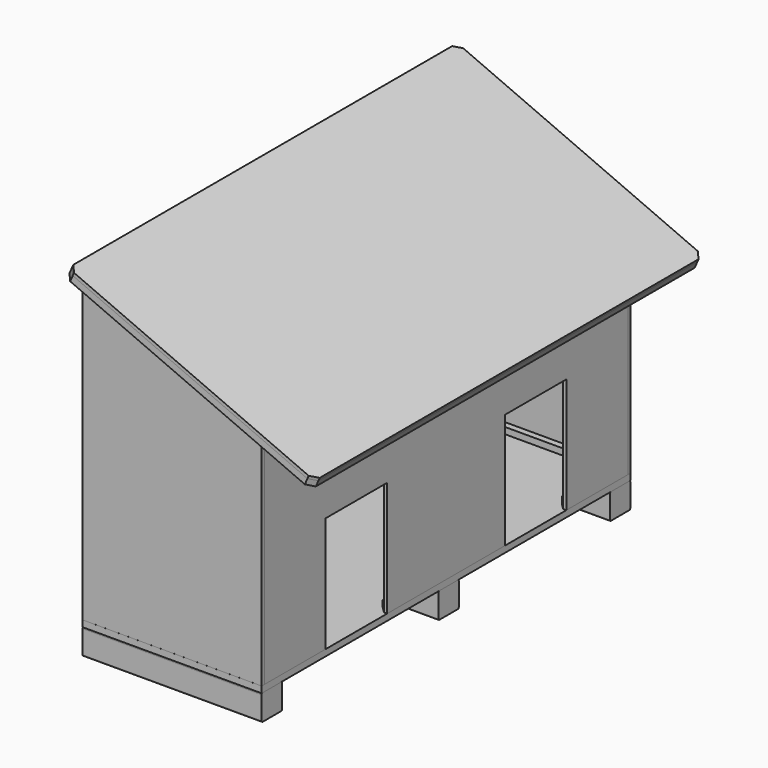
from build123d import *

# Parameters (mm, degrees)
F0_W      = 1803.4
F0_H      = 1219.2
F1_DEPTH  = 12.7
F3_DEPTH  = 12.7
F5_W      = 711.2
F5_H      = 1828.8
F6_DEPTH  = 25.4
F7_W      = 12.7
F7_H      = 901.7
F8_DEPTH  = 1803.4
F9_W      = 304.8
F9_H      = 457.2
F10_DEPTH = 12.7
F11_W     = 711.2
F11_H     = 101.6
F12_DEPTH = 101.6
F13_R     = 5.08
F16_W     = 25.4
F16_H     = 1219.2
F17_DEPTH = 25.4
F18_SIZE2 = 8.63599
F18_SIZE  = 25.39999
F20_W     = 1752.6
F20_H     = 25.4
F21_DEPTH = 25.4
F22_W     = 25.4
F22_H     = 927.1
F23_DEPTH = 25.4
F24_SIZE2 = 25.39999
F24_SIZE  = 8.63599
F26_W     = 279.4
F26_H     = 25.4
F27_DEPTH = 25.4
F28_SIZE  = 25.39999
F29_W     = 584.2
F29_H     = 25.4
F30_DEPTH = 25.4
F31_SIZE  = 25.39999
F32_W     = 279.4
F32_H     = 25.4
F33_DEPTH = 25.4
F34_SIZE  = 25.39999
F35_W     = 635
F35_H     = 25.4
F36_DEPTH = 25.4
F38_W     = 1066.8
F38_H     = 1930.4
F39_DEPTH = 12.7
F40_SIZE  = 25.4
F41_W     = 25.4
F41_H     = 1930.4
F42_DEPTH = 25.4
F43_SIZE  = 25.39999
F44_W     = 1041.4
F44_H     = 25.4
F45_DEPTH = 25.4
F46_SIZE  = 25.39999
F47_W     = 1041.4
F47_H     = 25.4
F48_DEPTH = 25.4
F49_SIZE  = 25.39999
F50_W     = 25.4
F50_H     = 1879.6
F51_DEPTH = 25.4
F53_DEPTH = 25.4
F55_W     = 101.6
F55_H     = 774.7
F56_DEPTH = 50.8


# Not quite as in the source:
# - a fillet or chamfer is up to 0.001 mm smaller than in the source, because OpenCascade refuses the exact size


with BuildPart() as f1:
    # F0 (on Right) → F1 (new body)
    with BuildSketch(Plane.YZ):
        with Locations((901.7, 609.6)):
            Rectangle(F0_W, F0_H)
    extrude(amount=F1_DEPTH)


with BuildPart() as f3:
    # F2 (on face) → F3 (new body)
    with BuildSketch(Plane(origin=(0, 1803.4, 0), x_dir=(-1, 0, 0), z_dir=(0, 1, 0))):
        Polygon((-711.2, 0), (0, 0), (0, 1219.2), (-12.7, 1219.2), (-711.2, 914.4), align=None)
    extrude(amount=F3_DEPTH)


with BuildPart() as f4_1:
    # F4: copy of F3
    add(f3.part.moved(Location((0, -1816.1, 0))))


with BuildPart() as f6:
    # F5 (on Top) → F6 (new body)
    with BuildSketch(Plane.XY):
        with Locations((355.6, 901.5832041594)):
            Rectangle(F5_W, F5_H)
    extrude(amount=-F6_DEPTH)


with BuildPart() as f8:
    # F7 (on face) → F8 (new body)
    with BuildSketch(Plane.XZ.offset(-1803.4)):
        with Locations((704.85, 450.85)):
            Rectangle(F7_W, F7_H)
    extrude(amount=F8_DEPTH)

    # F9 (on face) → F10 (cut)
    with BuildSketch(Plane.YZ.offset(711.2)):
        with Locations((457.2, 228.6)):
            Rectangle(F9_W, F9_H)
        with Locations((1346.2, 228.6)):
            Rectangle(F9_W, F9_H)
    extrude(amount=-F10_DEPTH, mode=Mode.SUBTRACT)


with BuildPart() as f12:
    # F11 (on face) → F12 (new body)
    with BuildSketch(Plane(origin=(0, 0, -25.4), x_dir=(1, 0, 0), z_dir=(0, 0, -1))):
        with Locations((355.6, -37.9832041594)):
            Rectangle(F11_W, F11_H)
    extrude(amount=F12_DEPTH)

    # F13
    f13_edges = [f12.edges().sort_by_distance(p)[0] for p in [
        (355.6, -12.816796, -127),
        (355.6, 88.783204, -127),
        (355.6, 88.783204, -25.4),
        (355.6, -12.816796, -25.4),
    ]]
    fillet(f13_edges, radius=F13_R)


with BuildPart() as f14_1:
    # F14: copy of F12
    add(f12.part.moved(Location((0, 876.3, 0))))


with BuildPart() as f15_1:
    # F15: copy of F12
    add(f12.part.moved(Location((0, 1727.2, 0))))


with BuildPart() as f17:
    # F16 (on face) → F17 (new body)
    with BuildSketch(Plane.YZ.offset(12.7)):
        with Locations((12.7, 609.6)):
            Rectangle(F16_W, F16_H)
    extrude(amount=F17_DEPTH)

    # F18 (size 25.4 and 8.636 in the source; OpenCascade refuses exactly that, so slightly less here)
    f18_edges = [f17.edges().sort_by_distance(p)[0] for p in [
        (38.1, 12.7, 1219.2),
    ]]
    f18_side = f17.faces().sort_by_distance((25.4, 12.7, 1219.2))[0]
    chamfer(f18_edges, length=F18_SIZE, length2=F18_SIZE2, reference=f18_side)


with BuildPart() as f19_1:
    # F19: copy of F17
    add(f17.part.moved(Location((0, 1778, 0))))


with BuildPart() as f21:
    # F20 (on face) → F21 (new body)
    with BuildSketch(Plane.YZ.offset(12.7)):
        with Locations((901.7, 12.7)):
            Rectangle(F20_W, F20_H)
    extrude(amount=F21_DEPTH)


with BuildPart() as f23:
    # F22 (on face) → F23 (new body)
    with BuildSketch(Plane(origin=(698.5, 0, 0), x_dir=(0, -1, 0), z_dir=(-1, 0, 0))):
        with Locations((-1790.7, 463.55)):
            Rectangle(F22_W, F22_H)
    extrude(amount=F23_DEPTH)

    # F24 (size 8.636 and 25.4 in the source; OpenCascade refuses exactly that, so slightly less here)
    f24_edges = [f23.edges().sort_by_distance(p)[0] for p in [
        (698.5, 1790.7, 927.1),
    ]]
    f24_side = f23.faces().sort_by_distance((698.5, 1790.7, 463.55))[0]
    chamfer(f24_edges, length=F24_SIZE, length2=F24_SIZE2, reference=f24_side)


with BuildPart() as f25_1:
    # F25: copy of F23
    add(f23.part.moved(Location((0, -1778, 0))))


with BuildPart() as f27:
    # F26 (on face) → F27 (new body)
    with BuildSketch(Plane(origin=(698.5, 0, 0), x_dir=(0, -1, 0), z_dir=(-1, 0, 0))):
        with Locations((-1638.3, 12.7)):
            Rectangle(F26_W, F26_H)
    extrude(amount=F27_DEPTH)

    # F28 (size 25.4 in the source; OpenCascade refuses exactly that, so slightly less here)
    f28_edges = [f27.edges().sort_by_distance(p)[0] for p in [
        (673.1, 1498.6, 12.7),
    ]]
    chamfer(f28_edges, length=F28_SIZE)


with BuildPart() as f30:
    # F29 (on face) → F30 (new body)
    with BuildSketch(Plane(origin=(698.5, 0, 0), x_dir=(0, -1, 0), z_dir=(-1, 0, 0))):
        with Locations((-901.7, 12.7)):
            Rectangle(F29_W, F29_H)
    extrude(amount=F30_DEPTH)

    # F31 (size 25.4 in the source; OpenCascade refuses exactly that, so slightly less here)
    f31_edges = [f30.edges().sort_by_distance(p)[0] for p in [
        (673.1, 1193.8, 12.7),
        (673.1, 609.6, 12.7),
    ]]
    chamfer(f31_edges, length=F31_SIZE)


with BuildPart() as f33:
    # F32 (on face) → F33 (new body)
    with BuildSketch(Plane(origin=(698.5, 0, 0), x_dir=(0, -1, 0), z_dir=(-1, 0, 0))):
        with Locations((-165.1, 12.7)):
            Rectangle(F32_W, F32_H)
    extrude(amount=F33_DEPTH)

    # F34 (size 25.4 in the source; OpenCascade refuses exactly that, so slightly less here)
    f34_edges = [f33.edges().sort_by_distance(p)[0] for p in [
        (673.1, 304.8, 12.7),
    ]]
    chamfer(f34_edges, length=F34_SIZE)


with BuildPart() as f36:
    # F35 (on face) → F36 (new body)
    with BuildSketch(Plane.XZ.offset(-1803.4)):
        with Locations((355.6, 12.7)):
            Rectangle(F35_W, F35_H)
    extrude(amount=F36_DEPTH)


with BuildPart() as f37_1:
    # F37: copy of F36
    add(f36.part.moved(Location((0, -1778, 0))))


with BuildPart() as f39:
    # F38 (on face) → F39 (new body)
    with BuildSketch(Plane(origin=(448.9472924188, 0, 1028.8375451264), x_dir=(0.9165393784, 0, -0.399944456), z_dir=(0.399944456, 0, 0.9165393784))):
        with Locations((20.3877192255, 901.7)):
            Rectangle(F38_W, F38_H)
    extrude(amount=F39_DEPTH)

    # F40
    f40_edges = [f39.edges().sort_by_distance(p)[0] for p in [
        (959.055192, -63.5, 813.173242),
        (959.055192, 1866.9, 813.173242),
        (-18.709017, 1866.9, 1239.833988),
        (-18.709017, -63.5, 1239.833988),
    ]]
    chamfer(f40_edges, length=F40_SIZE)


with BuildPart() as f42:
    # F41 (on face) → F42 (new body)
    with BuildSketch(Plane(origin=(448.9472924188, 0, 1028.8375451264), x_dir=(0.9165393784, 0, -0.399944456), z_dir=(-0.399944456, 0, -0.9165393784))):
        with Locations((-500.3122807745, -901.7)):
            Rectangle(F41_W, F41_H)
    extrude(amount=F42_DEPTH)

    # F43 (size 25.4 in the source; OpenCascade refuses exactly that, so slightly less here)
    f43_edges = [f42.edges().sort_by_distance(p)[0] for p in [
        (-26.327959, 1866.9, 1222.373913),
        (-26.327959, -63.5, 1222.373913),
    ]]
    chamfer(f43_edges, length=F43_SIZE)


with BuildPart() as f45:
    # F44 (on face) → F45 (new body)
    with BuildSketch(Plane(origin=(448.9472924188, 0, 1028.8375451264), x_dir=(0.9165393784, 0, -0.399944456), z_dir=(-0.399944456, 0, -0.9165393784))):
        with Locations((33.0877192255, -1854.2)):
            Rectangle(F44_W, F44_H)
    extrude(amount=F45_DEPTH)

    # F46 (size 25.4 in the source; OpenCascade refuses exactly that, so slightly less here)
    f46_edges = [f45.edges().sort_by_distance(p)[0] for p in [
        (951.43625, 1866.9, 795.713167),
    ]]
    chamfer(f46_edges, length=F46_SIZE)


with BuildPart() as f48:
    # F47 (on face) → F48 (new body)
    with BuildSketch(Plane(origin=(448.9472924188, 0, 1028.8375451264), x_dir=(0.9165393784, 0, -0.399944456), z_dir=(-0.399944456, 0, -0.9165393784))):
        with Locations((33.0877192255, 50.8)):
            Rectangle(F47_W, F47_H)
    extrude(amount=F48_DEPTH)

    # F49 (size 25.4 in the source; OpenCascade refuses exactly that, so slightly less here)
    f49_edges = [f48.edges().sort_by_distance(p)[0] for p in [
        (951.43625, -63.5, 795.713167),
    ]]
    chamfer(f49_edges, length=F49_SIZE)


with BuildPart() as f51:
    # F50 (on face) → F51 (new body)
    with BuildSketch(Plane(origin=(448.9472924188, 0, 1028.8375451264), x_dir=(0.9165393784, 0, -0.399944456), z_dir=(-0.399944456, 0, -0.9165393784))):
        with Locations((541.0877192255, -901.7)):
            Rectangle(F50_W, F50_H)
    extrude(amount=F51_DEPTH)


with BuildPart() as f53:
    # F52 (on face) → F53 (new body)
    with BuildSketch(Plane(origin=(0, 0, 0), x_dir=(-1, 0, 0), z_dir=(0, 1, 0))):
        Polygon((-673.1, 903.3125154187), (-38.1, 1180.4034245096), (-38.1, 1208.1163636364), (-673.1, 931.0254545455), align=None)
    extrude(amount=F53_DEPTH)


with BuildPart() as f54_1:
    # F54: copy of F53
    add(f53.part.moved(Location((0, 1778, 0))))


with BuildPart() as f56:
    # F55 (on face) → F56 (new body)
    with BuildSketch(Plane(origin=(0, 0, -25.4), x_dir=(1, 0, 0), z_dir=(0, 0, -1))):
        with Locations((495.3, -476.1332041594)):
            Rectangle(F55_W, F55_H)
    extrude(amount=F56_DEPTH)


with BuildPart() as f57_1:
    # F57: copy of F56
    add(f56.part.moved(Location((-279.4, 0, 0))))


with BuildPart() as f58_1:
    # F58: copy of F56
    add(f56.part.moved(Location((0, 863.6, 0))))


with BuildPart() as f59_1:
    # F59: copy of F57_1
    add(f57_1.part.moved(Location((0, 863.6, 0))))


solid = Compound([f1.part, f3.part, f4_1.part, f6.part, f8.part, f12.part, f14_1.part, f15_1.part, f17.part, f19_1.part, f21.part, f23.part, f25_1.part, f27.part, f30.part, f33.part, f36.part, f37_1.part, f39.part, f42.part, f45.part, f48.part, f51.part, f53.part, f54_1.part, f56.part, f57_1.part, f58_1.part, f59_1.part])
